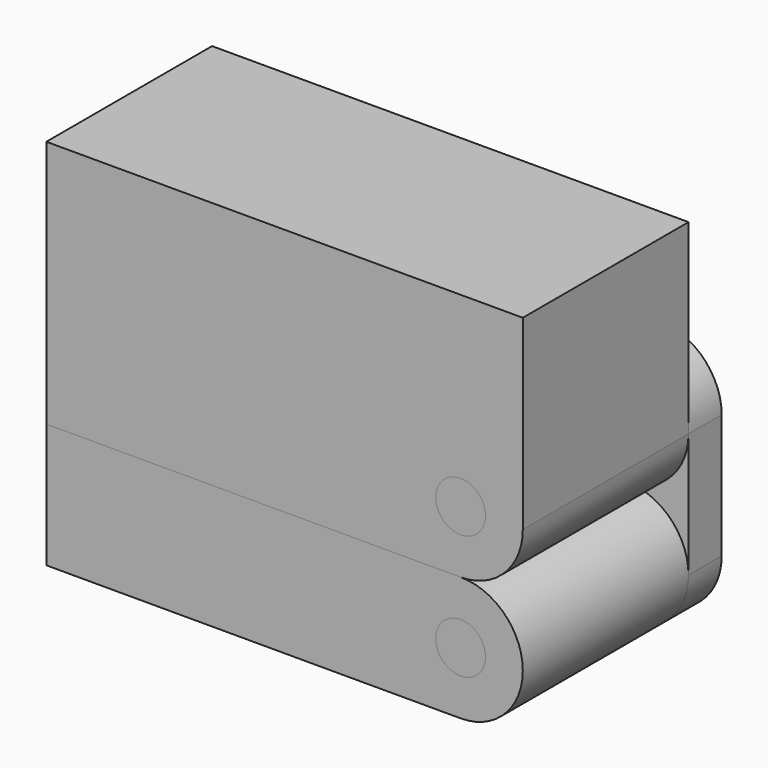
from build123d import *

# Parameters (mm, degrees)
F0_R     = 3
F1_DEPTH = 25
F2_DEPTH = 25
F3_DEPTH = 25
F5_DEPTH = 5


# Not quite as in the source:
# - a feature names something its author has since deleted; it is built from what else it names


with BuildPart() as f1:
    # F0 (on Front) → F1 (new body)
    with BuildSketch(Plane.XZ):
        with BuildLine():
            Line((-50, 0), (0, 0))
            ThreePointArc((0, 0), (5.3033008589, 2.1966991411), (7.5, 7.5))
            Line((7.5, 7.5), (7.5, 30))
            Line((7.5, 30), (-50, 30))
            Line((-50, 30), (-50, 15))
            Line((-50, 15), (-50, 0))
        make_face()
        with Locations((0, 7.5)):
            Circle(F0_R, mode=Mode.SUBTRACT)
    extrude(amount=F1_DEPTH)


with BuildPart() as f2:
    # F0 (on Front) → F2 (new body)
    with BuildSketch(Plane.XZ):
        with BuildLine():
            ThreePointArc((0, -15), (7.5, -7.5), (0, 0))
            Line((0, 0), (-50, 0))
            Line((-50, 0), (-50, -15))
            Line((-50, -15), (0, -15))
        make_face()
        with Locations((0, -7.5)):
            Circle(F0_R, mode=Mode.SUBTRACT)
    extrude(amount=F2_DEPTH)


with BuildPart() as f3:
    # F0 (on Front) → F3 (new body)
    with BuildSketch(Plane.XZ):
        with Locations((0, 7.5)):
            Circle(F0_R)
    extrude(amount=F3_DEPTH)



with BuildPart() as f3b:
    # F0 (on Front) → F3, piece 2 (new body)
    with BuildSketch(Plane.XZ):
        with Locations((0, -7.5)):
            Circle(F0_R)
    extrude(amount=F3_DEPTH)


with BuildPart() as f3_1:
    add(f3.part)

    add(f3b.part)  # F5 merges F3b
    # F4 (on Front) → F5 (join)
    with BuildSketch(Plane.XZ):
        with BuildLine():
            ThreePointArc((7.5, 7.5), (5.3033008589, 12.8033008589), (0, 15))
            ThreePointArc((0, 15), (-5.3033008589, 12.8033008589), (-7.5, 7.5))
            Line((-7.5, 7.5), (-7.5, -7.5))
            ThreePointArc((-7.5, -7.5), (-5.3033008589, -12.8033008589), (0, -15))
            ThreePointArc((0, -15), (5.3033008589, -12.8033008589), (7.5, -7.5))
            Line((7.5, -7.5), (7.5, 7.5))
        make_face()
    extrude(amount=-F5_DEPTH)


solid = Compound([f1.part, f2.part, f3_1.part])
